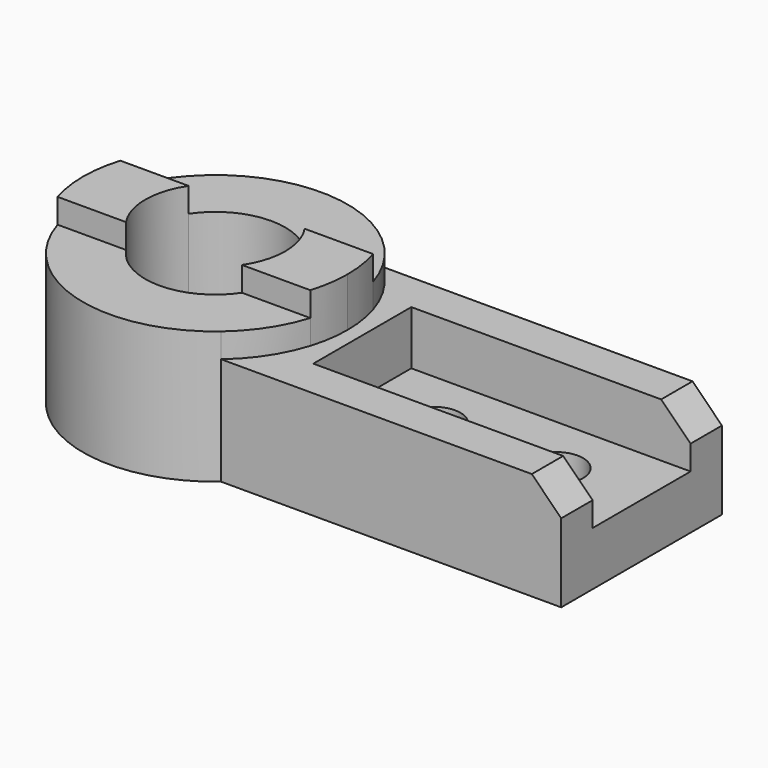
from build123d import *

# Parameters (mm, degrees)
F1_DEPTH = 44
F0_W     = 114
F0_H     = 50
F0_R     = 11.1
F2_DEPTH = 22
F3_DEPTH = 54
F4_DEPTH = 64
F6_DEPTH = 95.001


# Not quite as in the source:
# - a feature names something its author has since deleted; it is built from what else it names


with BuildPart() as f1:
    # F0 (on Top) → F1 (new body)
    with BuildSketch(Plane.XY):
        with BuildLine():
            ThreePointArc((51.5751878329, 16), (53.3903556037, 8.0913489921), (54, 0))
            ThreePointArc((54, 0), (53.3903556037, -8.0913489921), (51.5751878329, -16))
            ThreePointArc((51.5751878329, -16), (45.1247409006, -29.6607106903), (35.1425667816, -41))
            Line((35.1425667816, -41), (174, -41))
            Line((174, -41), (174, -25))
            Line((174, -25), (60, -25))
            Line((60, -25), (60, 25))
            Line((60, 25), (174, 25))
            Line((174, 25), (174, 41))
            Line((174, 41), (35.1425667816, 41))
            ThreePointArc((35.1425667816, 41), (45.1247409006, 29.6607106903), (51.5751878329, 16))
        make_face()
    extrude(amount=F1_DEPTH)

    # F0 (on Top) → F2 (join)
    with BuildSketch(Plane.XY):
        with Locations((117, 0)):
            Rectangle(F0_W, F0_H)
        with Locations((89, 0)):
            Circle(F0_R, mode=Mode.SUBTRACT)
        with Locations((139, 0)):
            Circle(F0_R, mode=Mode.SUBTRACT)
    extrude(amount=F2_DEPTH)

    # F0 (on Top) → F3 (join)
    with BuildSketch(Plane.XY):
        with BuildLine():
            ThreePointArc((35.1425667816, -41), (45.1247409006, -29.6607106903), (51.5751878329, -16))
            Line((51.5751878329, -16), (23.6755279772, -16))
            ThreePointArc((23.6755279772, -16), (0, -28.575), (-23.6755279772, -16))
            Line((-23.6755279772, -16), (-51.5751878329, -16))
            ThreePointArc((-51.5751878329, -16), (-14.9585346426, -51.8868214612), (35.1425667816, -41))
        make_face()
        with BuildLine():
            Line((23.6755279772, 16), (51.5751878329, 16))
            ThreePointArc((51.5751878329, 16), (45.1247409006, 29.6607106903), (35.1425667816, 41))
            ThreePointArc((35.1425667816, 41), (-14.9585346426, 51.8868214612), (-51.5751878329, 16))
            Line((-51.5751878329, 16), (-23.6755279772, 16))
            ThreePointArc((-23.6755279772, 16), (0, 28.575), (23.6755279772, 16))
        make_face()
    extrude(amount=F3_DEPTH)

    # F0 (on Top) → F4 (join)
    with BuildSketch(Plane.XY):
        with BuildLine():
            Line((-23.6755279772, 16), (-51.5751878329, 16))
            ThreePointArc((-51.5751878329, 16), (-54, 0), (-51.5751878329, -16))
            Line((-51.5751878329, -16), (-23.6755279772, -16))
            ThreePointArc((-23.6755279772, -16), (-28.575, 0), (-23.6755279772, 16))
        make_face()
        with BuildLine():
            ThreePointArc((51.5751878329, -16), (53.3903556037, -8.0913489921), (54, 0))
            ThreePointArc((54, 0), (53.3903556037, 8.0913489921), (51.5751878329, 16))
            Line((51.5751878329, 16), (23.6755279772, 16))
            ThreePointArc((23.6755279772, 16), (27.3226905424, 8.3666723687), (28.575, 0))
            ThreePointArc((28.575, 0), (27.3226905424, -8.3666723687), (23.6755279772, -16))
            Line((23.6755279772, -16), (51.5751878329, -16))
        make_face()
    extrude(amount=F4_DEPTH)

    # F5 (on face) → F6 (cut, through all)
    with BuildSketch(Plane.XZ.offset(41)):
        Polygon((174, 44), (162, 44), (174, 32), align=None)
    extrude(amount=-F6_DEPTH, mode=Mode.SUBTRACT)


solid = f1.part
